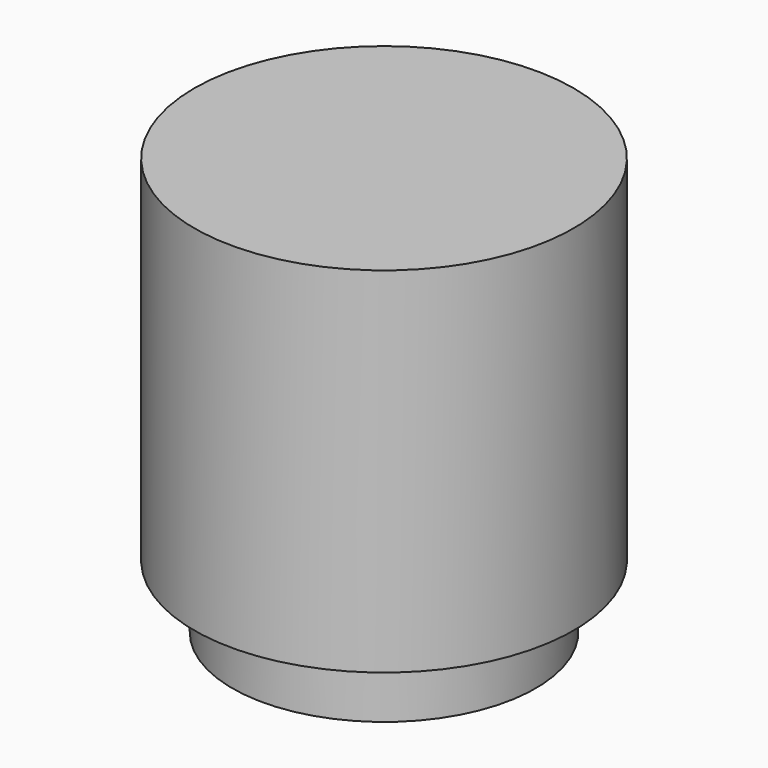
from build123d import *


# Not quite as in the source:
# - a feature names something its author has since deleted; it is built from what else it names


with BuildPart() as f1:
    # F0 (on Front) → F1 (revolve)
    with BuildSketch(Plane.XZ):
        with BuildLine():
            Line((-15, -28), (-12, -28))
            Line((-12, -28), (-12, -33))
            Line((-12, -33), (-9, -33))
            Line((-9, -33), (-9, -7.2415010072))
            ThreePointArc((-9, -7.2415010072), (-4.9914312836, -4.0779872119), (0, -3))
            Line((0, -3), (0, 0))
            Line((0, 0), (-15, 0))
            Line((-15, 0), (-15, -6))
            Line((-15, -6), (-15, -28))
        make_face()
    revolve(axis=Axis((0, 0, -1.5), (0, 0, -1)))


solid = f1.part
